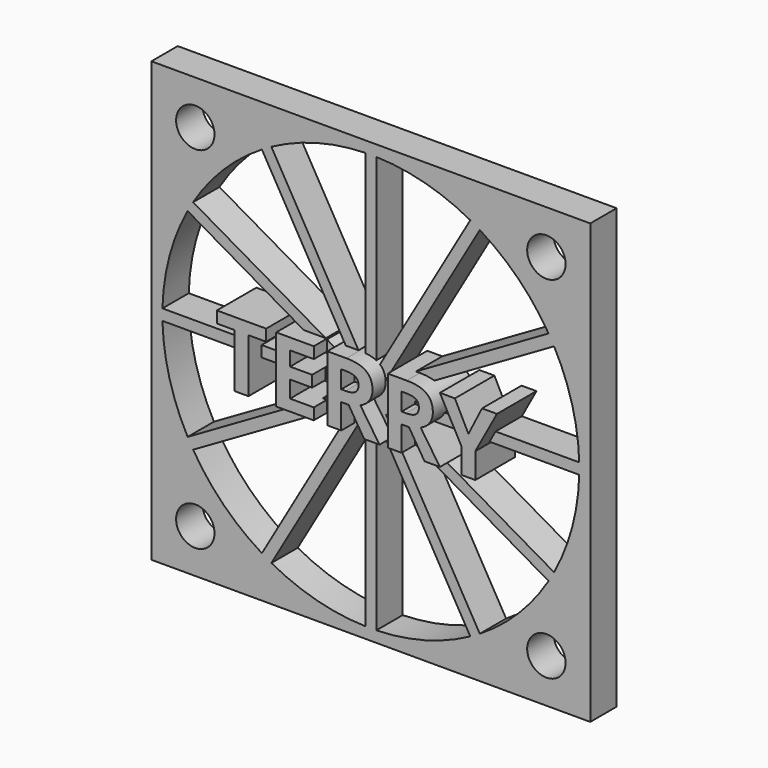
from build123d import *

# Parameters (mm, degrees)
F0_W         = 40
F0_H         = 40
F0_R         = 1.75
F1_DEPTH     = 3
F2_TEXT_SIZE = 8.3333333333
F3_DEPTH     = 4.5


# Not quite as in the source:
# - Text() gives the source's letters only with a copy of the font that has no kerning and outlines rounded to 1/6400 em; it was checked with that copy


with BuildPart() as f1:
    # F0 (on Front) → F1 (new body)
    with BuildSketch(Plane.XZ):
        Rectangle(F0_W, F0_H)
        with Locations((-16, -16)):
            Circle(F0_R, mode=Mode.SUBTRACT)
        with BuildLine():
            Line((-0.5, -1.8660254038), (-0.5, -18.9934199132))
            ThreePointArc((-0.5, -18.9934199132), (-4.9175618569, -18.3525906995), (-9.0636972547, -16.6987841496))
            Line((-9.0636972547, -16.6987841496), (-0.5, -1.8660254038))
        make_face(mode=Mode.SUBTRACT)
        with BuildLine():
            ThreePointArc((-16.6987841496, -9.0636972547), (-18.3525906995, -4.9175618569), (-18.9934199132, -0.5))
            Line((-18.9934199132, -0.5), (-1.8660254038, -0.5))
            Line((-1.8660254038, -0.5), (-16.6987841496, -9.0636972547))
        make_face(mode=Mode.SUBTRACT)
        with BuildLine():
            ThreePointArc((-9.9297226585, -16.1987841496), (-13.4350288425, -13.4350288425), (-16.1987841496, -9.9297226585))
            Line((-16.1987841496, -9.9297226585), (-1.3660254038, -1.3660254038))
            Line((-1.3660254038, -1.3660254038), (-9.9297226585, -16.1987841496))
        make_face(mode=Mode.SUBTRACT)
        with BuildLine():
            ThreePointArc((9.0636972547, -16.6987841496), (4.9175618569, -18.3525906995), (0.5, -18.9934199132))
            Line((0.5, -18.9934199132), (0.5, -1.8660254038))
            Line((0.5, -1.8660254038), (9.0636972547, -16.6987841496))
        make_face(mode=Mode.SUBTRACT)
        with Locations((16, -16)):
            Circle(F0_R, mode=Mode.SUBTRACT)
        with BuildLine():
            ThreePointArc((16.1987841496, -9.9297226585), (13.4350288425, -13.4350288425), (9.9297226585, -16.1987841496))
            Line((9.9297226585, -16.1987841496), (1.3660254038, -1.3660254038))
            Line((1.3660254038, -1.3660254038), (16.1987841496, -9.9297226585))
        make_face(mode=Mode.SUBTRACT)
        with BuildLine():
            ThreePointArc((18.9934199132, -0.5), (18.3525906995, -4.9175618569), (16.6987841496, -9.0636972547))
            Line((16.6987841496, -9.0636972547), (1.8660254038, -0.5))
            Line((1.8660254038, -0.5), (18.9934199132, -0.5))
        make_face(mode=Mode.SUBTRACT)
        with BuildLine():
            ThreePointArc((-18.9934199132, 0.5), (-18.3525906995, 4.9175618569), (-16.6987841496, 9.0636972547))
            Line((-16.6987841496, 9.0636972547), (-1.8660254038, 0.5))
            Line((-1.8660254038, 0.5), (-18.9934199132, 0.5))
        make_face(mode=Mode.SUBTRACT)
        with BuildLine():
            ThreePointArc((-16.1987841496, 9.9297226585), (-13.4350288425, 13.4350288425), (-9.9297226585, 16.1987841496))
            Line((-9.9297226585, 16.1987841496), (-1.3660254038, 1.3660254038))
            Line((-1.3660254038, 1.3660254038), (-16.1987841496, 9.9297226585))
        make_face(mode=Mode.SUBTRACT)
        with Locations((-16, 16)):
            Circle(F0_R, mode=Mode.SUBTRACT)
        with BuildLine():
            ThreePointArc((-9.0636972547, 16.6987841496), (-4.9175618569, 18.3525906995), (-0.5, 18.9934199132))
            Line((-0.5, 18.9934199132), (-0.5, 1.8660254038))
            Line((-0.5, 1.8660254038), (-9.0636972547, 16.6987841496))
        make_face(mode=Mode.SUBTRACT)
        with BuildLine():
            ThreePointArc((9.9297226585, 16.1987841496), (13.4350288425, 13.4350288425), (16.1987841496, 9.9297226585))
            Line((16.1987841496, 9.9297226585), (1.3660254038, 1.3660254038))
            Line((1.3660254038, 1.3660254038), (9.9297226585, 16.1987841496))
        make_face(mode=Mode.SUBTRACT)
        with BuildLine():
            ThreePointArc((16.6987841496, 9.0636972547), (18.3525906995, 4.9175618569), (18.9934199132, 0.5))
            Line((18.9934199132, 0.5), (1.8660254038, 0.5))
            Line((1.8660254038, 0.5), (16.6987841496, 9.0636972547))
        make_face(mode=Mode.SUBTRACT)
        with BuildLine():
            ThreePointArc((0.5, 18.9934199132), (4.9175618569, 18.3525906995), (9.0636972547, 16.6987841496))
            Line((9.0636972547, 16.6987841496), (0.5, 1.8660254038))
            Line((0.5, 1.8660254038), (0.5, 18.9934199132))
        make_face(mode=Mode.SUBTRACT)
        with Locations((16, 16)):
            Circle(F0_R, mode=Mode.SUBTRACT)
    extrude(amount=F1_DEPTH)

    # F2 (on Front) → F3 (join)
    with BuildSketch(Plane.XZ):
        with Locations((-13, -3)):
            Text('TERRY', F2_TEXT_SIZE, font='Open Sans', font_style=FontStyle.BOLD, text_align=(TextAlign.LEFT, TextAlign.BOTTOM))
    extrude(amount=F3_DEPTH)


solid = f1.part
